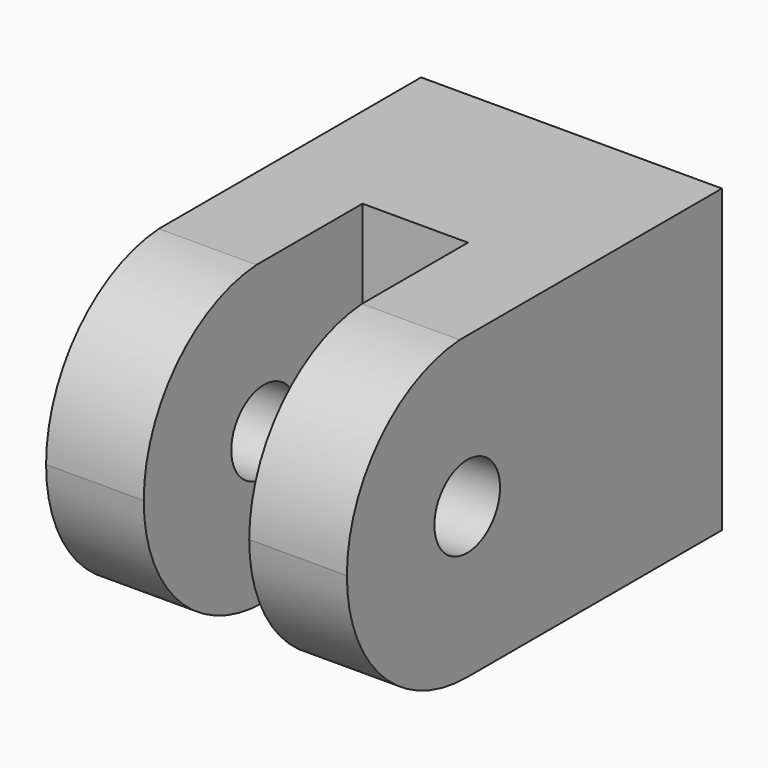
from build123d import *

# Parameters (mm, degrees)
F1_DEPTH = 7.7
F2_R     = 1.05
F3_DEPTH = 10


# Not quite as in the source:
# - ends of sketch curves that miss each other by under 0.0002 mm in the source are joined


with BuildPart() as f1:
    # F0 (on Top) → F1 (new body)
    with BuildSketch(Plane.XY):
        Polygon((3.85, 0), (0, 0), (-3.85, 0), (-3.85, -12), (-1.35, -12), (-1.35, -5), (0, -5), (1.35, -5), (1.35, -12), (3.85, -12), align=None)
    extrude(amount=F1_DEPTH)

    # F2 (on face) → F3 (cut)
    with BuildSketch(Plane(origin=(-3.85, 0, 0), x_dir=(0, -1, 0), z_dir=(-1, 0, 0))):
        with Locations((8.15, 3.85)):
            Circle(F2_R)
        with BuildLine():
            ThreePointArc((8.3927668004, 7.7), (10.9570802224, 6.4904376141), (12.0000020258, 3.8539515808))
            Line((12.0000020258, 3.8539515808), (12, 7.7))
            Line((12, 7.7), (8.3927668004, 7.7))
        make_face()
        with BuildLine():
            ThreePointArc((12.0000020258, 3.8539515808), (10.8726018857, 1.1301923043), (8.15, 0))
            Line((8.15, 0), (12, 0))
            Line((12, 0), (12.0000020258, 3.8539515808))
        make_face()
    extrude(amount=-F3_DEPTH, mode=Mode.SUBTRACT)


solid = f1.part
